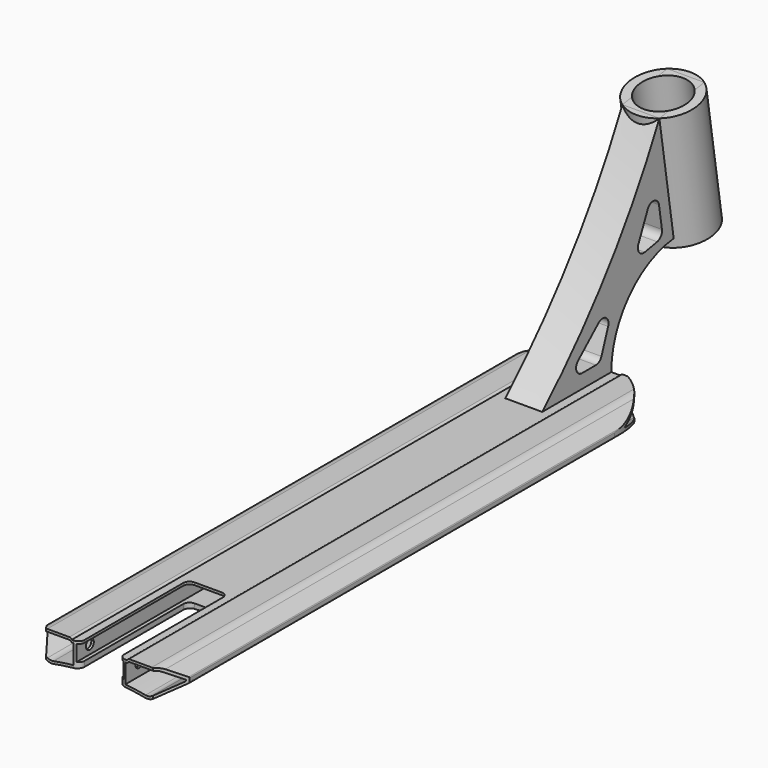
from build123d import *

# Parameters (mm, degrees)
F1_DEPTH         = 250
F2_W             = 38
F2_H             = 13
F3_DEPTH         = 250
F4_T1_DEPTH      = 509.3674969976
F5_R             = 9
F6_R             = 1
F8_DEPTH         = 500.001
F10_DEPTH        = 4.1102345884
F10_DEPTH_BACK   = 19.4100705928
F12_DEPTH        = 19.4100706928
F12_DEPTH_BACK   = 4.1102347011
F13_F1_R         = 4.9999
F13_F2_R         = 5
F13_F3_R         = 5
F13_F4_R         = 4.9999
F13_F5_R         = 5
F13_F6_R         = 5
F16_D            = 8
F16_DEPTH        = 12
F16_TIP          = 2.4034424761
F16_ON_F15_D     = 8
F16_ON_F15_DEPTH = 12
F16_ON_F15_TIP   = 2.4034424761
F18_DEPTH        = 15
F19_R            = 27.5
F20_DEPTH        = 100
F22_D            = 40
F24_DEPTH        = 72.5010001
F25_R            = 6


# Not quite as in the source:
# - a fillet or chamfer that OpenCascade refuses, or shapes differently, is made with other operations: its cross-section is extruded or revolved along the edge and cut away or added
# - a fillet or chamfer is up to 0.001 mm smaller than in the source, because OpenCascade refuses the exact size


with BuildPart() as f1:
    # F0 (on Front) → F1 (new body, symmetric)
    with BuildSketch(Plane.XZ):
        with BuildLine():
            Line((22.5, 18.1090705928), (0, 18.1090705928))
            Line((0, 18.1090705928), (-22.5, 18.1090705928))
            Line((-22.5, 18.1090705928), (-22.5, 19.4090705928))
            Line((-22.5, 19.4090705928), (-45.5824640741, 19.4090705928))
            Line((-45.5824640741, 19.4090705928), (-57.5, 9.4090705928))
            Line((-57.5, 9.4090705928), (-57.5, 5.4090705928))
            Line((-57.5, 5.4090705928), (-40.1794919243, -4.5909294072))
            ThreePointArc((-40.1794919243, -4.5909294072), (0, -0.5133845487), (40.1794919243, -4.5909294072))
            Line((40.1794919243, -4.5909294072), (57.5, 5.4090705928))
            Line((57.5, 5.4090705928), (57.5, 9.4090705928))
            Line((57.5, 9.4090705928), (45.5824640741, 19.4090705928))
            Line((45.5824640741, 19.4090705928), (22.5, 19.4090705928))
            Line((22.5, 19.4090705928), (22.5, 18.1090705928))
        make_face()
    extrude(amount=F1_DEPTH, both=True)

    # F2 (on Front) → F3 (cut, symmetric)
    with BuildSketch(Plane.XZ):
        with Locations((0, 9.6090705928)):
            Rectangle(F2_W, F2_H)
    extrude(amount=F3_DEPTH, both=True, mode=Mode.SUBTRACT)

    # F4: fillet of radius 2 on 2 edges, made by hand

    # F4_s2 → F4_t1 (cut)
    with BuildSketch(Plane.XZ.offset(-254.6837484988)):
        with BuildLine():
            ThreePointArc((-22.5, 18.1090705928), (-23.2333239744, 19.0522382654), (-24.3734993995, 19.4090705928))
            Line((-24.3734993995, 19.4090705928), (-22.5, 19.4090705928))
            Line((-22.5, 19.4090705928), (-22.5, 18.1090705928))
        make_face()
        with BuildLine():
            ThreePointArc((24.3734993995, 19.4090705928), (23.2333239744, 19.0522382654), (22.5, 18.1090705928))
            Line((22.5, 18.1090705928), (22.5, 19.4090705928))
            Line((22.5, 19.4090705928), (24.3734993995, 19.4090705928))
        make_face()
    extrude(amount=F4_T1_DEPTH, mode=Mode.SUBTRACT)

    # F5
    f5_edges = [f1.edges().sort_by_distance(p)[0] for p in [
        (-45.582464, 0, 19.409071),
        (45.582464, 0, 19.409071),
        (40.179492, 0, -4.590929),
        (-40.179492, 0, -4.590929),
    ]]
    fillet(f5_edges, radius=F5_R)

    # F6
    f6_edges = [f1.edges().sort_by_distance(p)[0] for p in [
        (57.5, 0, 9.409071),
        (57.5, 0, 5.409071),
        (-57.5, 0, 5.409071),
        (-57.5, 0, 9.409071),
    ]]
    fillet(f6_edges, radius=F6_R)

    # F7 (on face) → F8 (cut, through all)
    with BuildSketch(Plane.XZ.offset(250)):
        with BuildLine():
            Line((21, 16.1090705928), (21, 3.1090705928))
            Line((21, 3.1090705928), (21, 0.3920658502))
            ThreePointArc((21, 0.3920658502), (29.1789785809, -0.6319516717), (37.3093701274, -1.9887994196))
            ThreePointArc((37.3093701274, -1.9887994196), (39.7790673433, -2.0096074679), (42.1022690923, -1.1714124149))
            Line((42.1022690923, -1.1714124149), (55.6135241478, 6.6293143285))
            ThreePointArc((55.6135241478, 6.6293143285), (56.1097188459, 7.4081839895), (55.7563117574, 8.2613841754))
            Line((55.7563117574, 8.2613841754), (46.8062452335, 15.7713816947))
            ThreePointArc((46.8062452335, 15.7713816947), (44.7008729689, 16.9869189383), (42.3067319657, 17.4090705928))
            Line((42.3067319657, 17.4090705928), (24.3734993995, 17.4090705928))
            ThreePointArc((24.3734993995, 17.4090705928), (23.2333239744, 17.0522382654), (22.5, 16.1090705928))
            Line((22.5, 16.1090705928), (21, 16.1090705928))
        make_face()
        with BuildLine():
            ThreePointArc((-42.1022690923, -1.1714124149), (-39.7790673433, -2.0096074679), (-37.3093701274, -1.9887994196))
            ThreePointArc((-37.3093701274, -1.9887994196), (-29.1789785809, -0.6319516717), (-21, 0.3920658502))
            Line((-21, 0.3920658502), (-21, 3.1090705928))
            Line((-21, 3.1090705928), (-21, 16.1090705928))
            Line((-21, 16.1090705928), (-22.5, 16.1090705928))
            ThreePointArc((-22.5, 16.1090705928), (-23.2333239744, 17.0522382654), (-24.3734993995, 17.4090705928))
            Line((-24.3734993995, 17.4090705928), (-42.3067319657, 17.4090705928))
            ThreePointArc((-42.3067319657, 17.4090705928), (-44.7008729689, 16.9869189383), (-46.8062452335, 15.7713816947))
            Line((-46.8062452335, 15.7713816947), (-55.7563117574, 8.2613841754))
            ThreePointArc((-55.7563117574, 8.2613841754), (-56.1097188459, 7.4081839895), (-55.6135241478, 6.6293143285))
            Line((-55.6135241478, 6.6293143285), (-42.1022690923, -1.1714124149))
        make_face()
    extrude(amount=-F8_DEPTH, mode=Mode.SUBTRACT)

    # F9 (on Top) → F10 (cut, two sides)
    with BuildSketch(Plane.XY) as f10_sk:
        with BuildLine():
            ThreePointArc((-57.5, 200), (0, 257.5), (57.5, 200))
            Line((57.5, 200), (57.5, 280))
            Line((57.5, 280), (-57.5, 280))
            Line((-57.5, 280), (-57.5, 200))
        make_face()
    extrude(amount=-F10_DEPTH, mode=Mode.SUBTRACT)
    extrude(f10_sk.sketch, amount=F10_DEPTH_BACK, mode=Mode.SUBTRACT)

    # F11 (on Top) → F12 (cut, two sides)
    with BuildSketch(Plane.XY) as f12_sk:
        Polygon((-43.2975540478, -250), (-68, -216), (-68, -346), (68, -346), (68, -216), (43.2975540478, -250), (16, -250), (16, -140), (-16, -140), (-16, -250), align=None)
    extrude(amount=F12_DEPTH, mode=Mode.SUBTRACT)
    extrude(f12_sk.sketch, amount=-F12_DEPTH_BACK, mode=Mode.SUBTRACT)

    # F13: fillet of radius 5 on 8 edges, made by hand

    # F13_f1 (radius 5 in the source; OpenCascade refuses exactly that, so slightly less here)
    f13_f1_edges = [f1.edges().sort_by_distance(p)[0] for p in [
        (16, -250, 0.9773293771),
    ]]
    fillet(f13_f1_edges, radius=F13_F1_R)

    # F13_f2
    f13_f2_edges = [f1.edges().sort_by_distance(p)[0] for p in [
        (16, -140, 0.9773293771),
    ]]
    fillet(f13_f2_edges, radius=F13_F2_R)

    # F13_f3
    f13_f3_edges = [f1.edges().sort_by_distance(p)[0] for p in [
        (16, -140, 17.1090705928),
    ]]
    fillet(f13_f3_edges, radius=F13_F3_R)

    # F13_f4 (radius 5 in the source; OpenCascade refuses exactly that, so slightly less here)
    f13_f4_edges = [f1.edges().sort_by_distance(p)[0] for p in [
        (-16, -250, 17.1090705928),
    ]]
    fillet(f13_f4_edges, radius=F13_F4_R)

    # F13_f5
    f13_f5_edges = [f1.edges().sort_by_distance(p)[0] for p in [
        (-16, -140, 0.9773293771),
    ]]
    fillet(f13_f5_edges, radius=F13_F5_R)

    # F13_f6
    f13_f6_edges = [f1.edges().sort_by_distance(p)[0] for p in [
        (-16, -140, 17.1090705928),
    ]]
    fillet(f13_f6_edges, radius=F13_F6_R)

    # F16 (one way)
    with BuildSketch(Plane.YZ.offset(21)):
        with Locations((-236, 10.3920658502)):
            Circle(F16_D / 2)
    extrude(amount=-F16_DEPTH, mode=Mode.SUBTRACT)
    with Locations(Plane.YZ.offset(21)):
        with Locations((-236, 10.3920658502)):
            with Locations((0, 0, -(F16_DEPTH + F16_TIP / 2))):  # 118° drill point
                Cone(0, F16_D / 2, F16_TIP, mode=Mode.SUBTRACT)

    # F16 on F15 (one way)
    with BuildSketch(Plane(origin=(-21, 0, 0), x_dir=(0, -1, 0), z_dir=(-1, 0, 0))):
        with Locations((236, 10.3920658502)):
            Circle(F16_ON_F15_D / 2)
    extrude(amount=-F16_ON_F15_DEPTH, mode=Mode.SUBTRACT)
    with Locations(Plane(origin=(-21, 0, 0), x_dir=(0, -1, 0), z_dir=(-1, 0, 0))):
        with Locations((236, 10.3920658502)):
            with Locations((0, 0, -(F16_ON_F15_DEPTH + F16_ON_F15_TIP / 2))):  # 118° drill point
                Cone(0, F16_ON_F15_D / 2, F16_ON_F15_TIP, mode=Mode.SUBTRACT)

    # F17 (on Right) → F18 (join, symmetric)
    with BuildSketch(Plane.YZ):
        with BuildLine():
            ThreePointArc((298.7642824058, 179.4090705928), (246.7870939845, 93.3068455255), (180, 18.1090705928))
            Line((180, 18.1090705928), (250, 18.1090705928))
            ThreePointArc((250, 18.1090705928), (268.1797502143, 65.1692630292), (313.2760489184, 87.7853827933))
            Line((313.2760489184, 87.7853827933), (314.4077289098, 80.6402365333))
            Line((314.4077289098, 80.6402365333), (359.8413925772, 87.8362219252))
            Line((359.8413925772, 87.8362219252), (344.1979460732, 186.6050559847))
            Line((344.1979460732, 186.6050559847), (298.7642824058, 179.4090705928))
        make_face()
    extrude(amount=F18_DEPTH, both=True)

    # F19 (on face) → F20 (join, through all)
    with BuildSketch(Plane(origin=(0, -20.4089434853, 128.8569978435), x_dir=(1, 0, 0), z_dir=(0, -0.156434465, 0.9876883406))):
        with Locations((0, 346.1517603)):
            Circle(F19_R)
    extrude(amount=-F20_DEPTH)

    # F22 (through all)
    with Locations(Plane(origin=(0, -20.4089434853, 128.8569978435), x_dir=(1, 0, 0), z_dir=(0, -0.156434465, 0.9876883406))):
        with Locations((0, 346.1517603)):
            Hole(F22_D / 2)

    # F23 (on face) → F24 (cut, through all)
    with BuildSketch(Plane.YZ.offset(15)):
        Polygon((254.9629461589, 74.4090705928), (204.5842856169, 29.4090705928), (238.5842856169, 29.4090705928), align=None)
        Polygon((302.232862731, 93.272441523), (295.1933118042, 137.7184168498), (272.7398063184, 87.7806637196), align=None)
    extrude(amount=-F24_DEPTH, mode=Mode.SUBTRACT)

    # F25
    f25_edges = [f1.edges().sort_by_distance(p)[0] for p in [
        (0, 295.193312, 137.718417),
        (0, 272.739806, 87.780664),
        (0, 302.232863, 93.272442),
        (0, 254.962946, 74.409071),
        (0, 204.584286, 29.409071),
        (0, 238.584286, 29.409071),
    ]]
    fillet(f25_edges, radius=F25_R)


solid = f1.part
